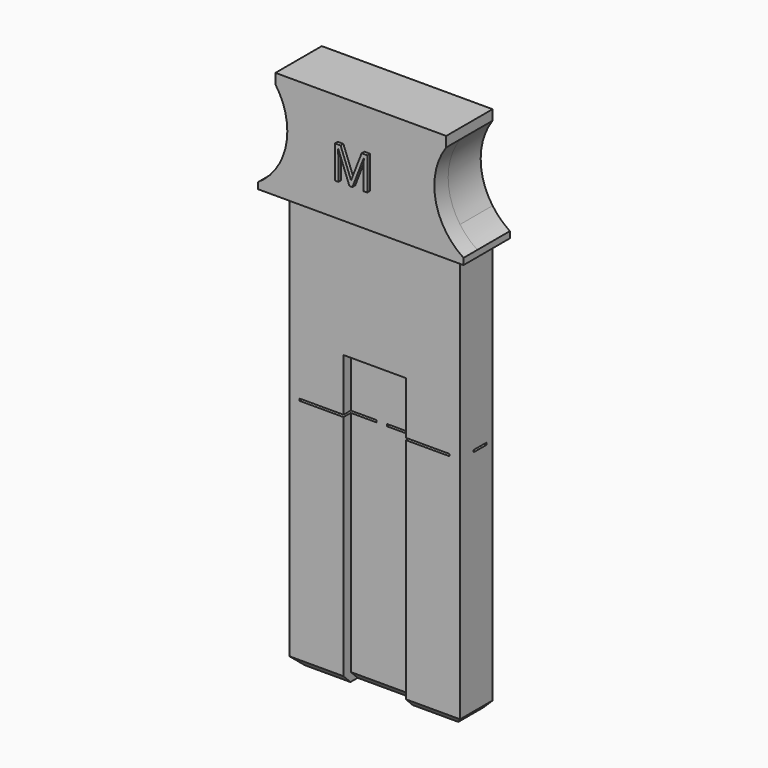
from build123d import *

# Parameters (mm, degrees)
F0_W          = 1.2
F0_H          = 0.24
F1_DEPTH      = 4.7
F3_DEPTH      = 1.05
F6_DEPTH      = 2
F7_SIZE       = 1
F8_W          = 1.85
F8_H          = 0.24
F9_DEPTH      = 125
F10_TEXT_SIZE = 5.3085904155
F11_DEPTH     = 0.4


# Not quite as in the source:
# - Text() gives the source's letters only with a copy of the font that has no kerning and outlines rounded to 1/6400 em; it was checked with that copy


with BuildPart() as f1:
    # F0 (on Front) → F1 (new body)
    with BuildSketch(Plane.XZ):
        with BuildLine():
            Line((0, 27.38), (0, 0))
            Line((0, 0), (19.75, 0))
            Line((19.75, 0), (19.75, 27.38))
            Line((19.75, 27.38), (18.55, 27.38))
            Line((18.55, 27.38), (10.475, 27.38))
            Line((10.475, 27.38), (10.475, 27.62))
            Line((10.475, 27.62), (18.55, 27.62))
            Line((18.55, 27.62), (19.75, 27.62))
            Line((19.75, 27.62), (19.75, 48.7))
            Line((19.75, 48.7), (19.75, 51.3716775767))
            ThreePointArc((19.75, 51.3716775767), (18.375, 55.7), (19.75, 60.0283224233))
            Line((19.75, 60.0283224233), (19.75, 61.2))
            Line((19.75, 61.2), (0, 61.2))
            Line((0, 61.2), (0, 60.0283224233))
            ThreePointArc((0, 60.0283224233), (1.0229892277, 57.9707377656), (1.375, 55.7))
            ThreePointArc((1.375, 55.7), (1.0229892277, 53.4292622344), (0, 51.3716775767))
            Line((0, 51.3716775767), (0, 48.7))
            Line((0, 48.7), (0, 27.62))
            Line((0, 27.62), (1.2, 27.62))
            Line((1.2, 27.62), (9.275, 27.62))
            Line((9.275, 27.62), (9.275, 27.38))
            Line((9.275, 27.38), (1.2, 27.38))
            Line((1.2, 27.38), (0, 27.38))
        make_face()
        with BuildLine():
            Line((-2, 48.7), (0, 48.7))
            Line((0, 48.7), (0, 51.3716775767))
            ThreePointArc((0, 51.3716775767), (-0.9094386331, 50.3103878035), (-2, 49.4362650918))
            Line((-2, 49.4362650918), (-2, 48.7))
        make_face()
        with BuildLine():
            Line((19.75, 51.3716775767), (19.75, 48.7))
            Line((19.75, 48.7), (21.75, 48.7))
            Line((21.75, 48.7), (21.75, 49.4362650918))
            ThreePointArc((21.75, 49.4362650918), (20.6594386331, 50.3103878035), (19.75, 51.3716775767))
        make_face()
        with Locations((0.6, 27.5)):
            Rectangle(F0_W, F0_H)
        with Locations((19.15, 27.5)):
            Rectangle(F0_W, F0_H)
    extrude(amount=F1_DEPTH)

    # F2 (on face) → F3 (cut)
    with BuildSketch(Plane.XZ.offset(4.7)):
        Polygon((13.475, 33.7), (6.275, 33.7), (6.275, 2.2), (6.275, 0), (13.475, 0), (13.475, 2.2), align=None)
    extrude(amount=-F3_DEPTH, mode=Mode.SUBTRACT)

    # F5 (on face) → F6 (join)
    with BuildSketch(Plane.XZ.offset(4.7)):
        with BuildLine():
            Line((-2, 48.7), (0, 48.7))
            Line((0, 48.7), (19.75, 48.7))
            Line((19.75, 48.7), (21.75, 48.7))
            Line((21.75, 48.7), (21.75, 49.4362650918))
            ThreePointArc((21.75, 49.4362650918), (18.5052276407, 54.3084342015), (19.75, 60.0283224233))
            Line((19.75, 60.0283224233), (19.75, 61.2))
            Line((19.75, 61.2), (0, 61.2))
            Line((0, 61.2), (0, 60.0283224233))
            ThreePointArc((0, 60.0283224233), (1.2447723593, 54.3084342015), (-2, 49.4362650918))
            Line((-2, 49.4362650918), (-2, 48.7))
        make_face()
    extrude(amount=F6_DEPTH)

    # F7
    f7_edges = [f1.edges().sort_by_distance(p)[0] for p in [
        (0, -2.35, 0),
        (19.75, -2.35, 0),
        (3.1375, -4.7, 0),
        (16.6125, -4.7, 0),
        (9.875, -3.65, 0),
    ]]
    chamfer(f7_edges, length=F7_SIZE)

    # F8 (on face) → F9 (cut, symmetric)
    with BuildSketch(Plane(origin=(9.275, 0, 0), x_dir=(0, -1, 0), z_dir=(-1, 0, 0))):
        with Locations((1.825, 27.5)):
            Rectangle(F8_W, F8_H)
    extrude(amount=F9_DEPTH, both=True, mode=Mode.SUBTRACT)

    # F10 (on face) → F11 (join)
    with BuildSketch(Plane.XZ.offset(6.7)):
        with Locations((6.6712992266, 52.7323260903)):
            Text('M', F10_TEXT_SIZE, font='Open Sans', text_align=(TextAlign.LEFT, TextAlign.BOTTOM))
    extrude(amount=F11_DEPTH)


solid = f1.part
